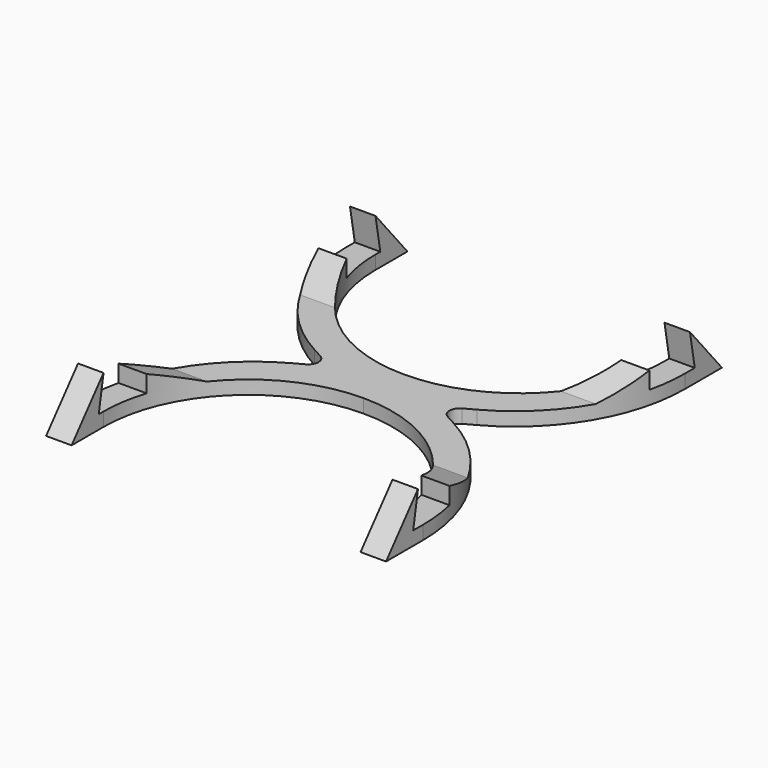
from build123d import *

# Parameters (mm, degrees)
F1_DEPTH = 50
F4_DEPTH = 14.001
F6_DEPTH = 4
F7_R     = 50
F8_R     = 3


# Not quite as in the source:
# - a pattern or mirror of a feature is missing from the dataset's text; its kind, count and spacing are read off the source's solid


with BuildPart() as f1:
    # F0 (on Right) → F1 (new body, symmetric)
    with BuildSketch(Plane.YZ):
        Polygon((0, 4), (0, 0), (61.7473948365, 0), (50, 14), (51.7632698071, 4), (36.7632698071, 4), (36.7632698071, 9), (23.5265396142, 4), align=None)
    extrude(amount=F1_DEPTH, both=True)

    # F2: F1 across face


with BuildPart() as f1_1:
    add(f1.part)
    add(f1.part.mirror(Plane(origin=(0, 0, 2), x_dir=(1, 0, 0), z_dir=(0, -1, 0))))

    # F3 (on face) → F4 (cut, through all)
    with BuildSketch(Plane(origin=(0, 0, 0), x_dir=(1, 0, 0), z_dir=(0, 0, -1))):
        with BuildLine():
            Line((42.5, 50), (42.5, 61.7473948365))
            Line((42.5, 61.7473948365), (0, 61.7473948365))
            Line((0, 61.7473948365), (-42.5, 61.7473948365))
            Line((-42.5, 61.7473948365), (-42.5, 50))
            ThreePointArc((-42.5, 50), (-30.0520382004, 19.9479617996), (0, 7.5))
            ThreePointArc((0, 7.5), (30.0520382004, 19.9479617996), (42.5, 50))
        make_face()
    f4 = extrude(amount=-F4_DEPTH, mode=Mode.SUBTRACT)

    # F4_copies: F4 across plane
    add(f4.mirror(Plane.ZX), mode=Mode.SUBTRACT)

    # F5 (on face) → F6 (cut, through all)
    with BuildSketch(Plane.XY.offset(4)):
        Polygon((-50, 18.5265396142), (-50, -18.5265396142), (-16.0078105936, 0), align=None)
        Polygon((50, 18.5265396142), (16.0078105936, 0), (50, -18.5265396142), align=None)
    extrude(amount=-F6_DEPTH, mode=Mode.SUBTRACT)

    # F7
    f7_edges = [f1_1.edges().sort_by_distance(p)[0] for p in [
        (50, -18.52654, 2),
        (50, 18.52654, 2),
        (-50, -18.52654, 2),
        (-50, 18.52654, 2),
    ]]
    fillet(f7_edges, radius=F7_R)

    # F8
    f8_edges = [f1_1.edges().sort_by_distance(p)[0] for p in [
        (-16.007811, 0, 2),
        (16.007811, 0, 2),
    ]]
    fillet(f8_edges, radius=F8_R)


solid = f1_1.part
